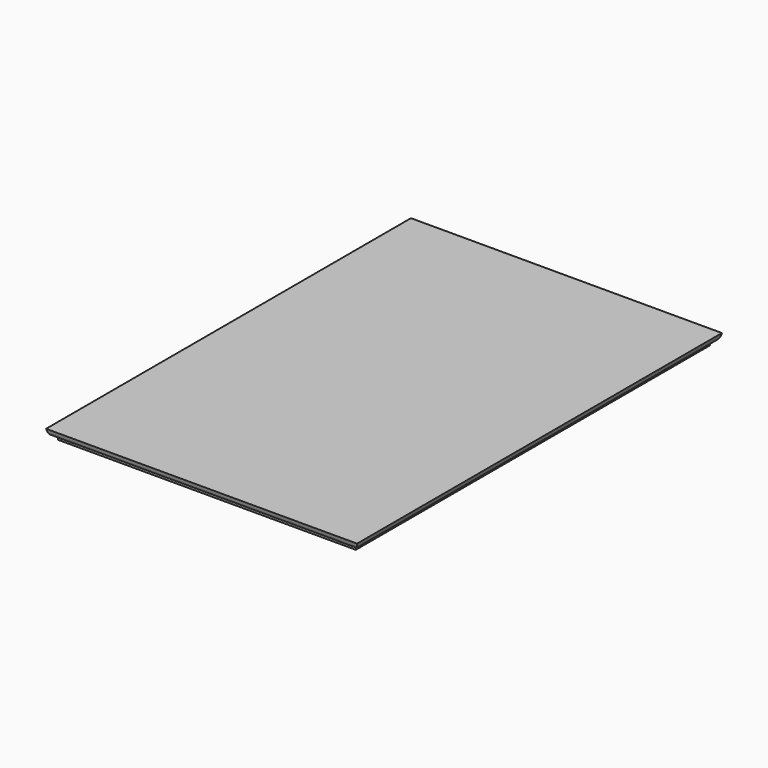
from build123d import *

# Parameters (mm, degrees)
F0_W     = 1524
F0_H     = 2235.2
F1_DEPTH = 50.8
F2_W     = 76.2
F2_H     = 50.8
F3_DEPTH = 12.7
F6_DEPTH = 1524.001
F7_DEPTH = 2235.201


with BuildPart() as f1:
    # F0 (on Top) → F1 (new body)
    with BuildSketch(Plane.XY):
        Rectangle(F0_W, F0_H)
    extrude(amount=F1_DEPTH)

    # F2 (on face) → F3 (cut)
    with BuildSketch(Plane(origin=(0, 0, 0), x_dir=(1, 0, 0), z_dir=(0, 0, -1))):
        with Locations((622.3, 914.4)):
            Rectangle(F2_W, F2_H)
        Polygon((584.2, 939.8), (660.4, 939.8), (660.4, 889), (685.8, 889), (685.8, 990.6), (584.2, 990.6), align=None)
        Polygon((584.2, 889), (584.2, 939.8), (-584.2, 939.8), (-584.2, 889), (-660.4, 889), (-660.4, -889), (-584.2, -889), (-584.2, -939.8), (584.2, -939.8), (584.2, -889), (660.4, -889), (660.4, 889), align=None)
        with Locations((-622.3, 914.4)):
            Rectangle(F2_W, F2_H)
        Polygon((-660.4, 939.8), (-584.2, 939.8), (-584.2, 990.6), (-685.8, 990.6), (-685.8, 889), (-660.4, 889), align=None)
        Polygon((685.8, -889), (660.4, -889), (660.4, -939.8), (584.2, -939.8), (584.2, -990.6), (685.8, -990.6), align=None)
        with Locations((622.3, -914.4)):
            Rectangle(F2_W, F2_H)
        with Locations((-622.3, -914.4)):
            Rectangle(F2_W, F2_H)
        Polygon((-660.4, -939.8), (-660.4, -889), (-685.8, -889), (-685.8, -990.6), (-584.2, -990.6), (-584.2, -939.8), align=None)
    extrude(amount=-F3_DEPTH, mode=Mode.SUBTRACT)

    # F5 (on face) → F6 (cut, through all)
    with BuildSketch(Plane(origin=(-762, 0, 0), x_dir=(0, -1, 0), z_dir=(-1, 0, 0))):
        with BuildLine():
            add(Edge.make_bspline(
                [(-1117.6, 50.8), (-1115.659954, 41.521689), (-1111.224864, 23.411832), (-1093.611323, 16.951729), (-1084.674984, 13.955233)],
                knots=[0, 0, 0, 0, 0.499842, 1, 1, 1, 1], degree=3))
            Line((-1117.6, 50.8), (-1117.6, 0))
            Line((-1117.6, 0), (-1084.674984, 0))
            Line((-1084.674984, 0), (-1084.674984, 13.955233))
        make_face()
        with BuildLine():
            Line((1117.6, 0), (1117.6, 50.8))
            add(Edge.make_bspline(
                [(1117.6, 50.8), (1115.659954, 41.521689), (1111.224864, 23.411832), (1093.611323, 16.951729), (1084.674984, 13.955233)],
                knots=[0, 0, 0, 0, 0.499842, 1, 1, 1, 1], degree=3))
            Line((1084.674984, 13.955233), (1084.674984, 0))
            Line((1084.674984, 0), (1117.6, 0))
        make_face()
    extrude(amount=-F6_DEPTH, mode=Mode.SUBTRACT)

    # F4 (on face) → F7 (cut, through all)
    with BuildSketch(Plane(origin=(0, 1117.6, 0), x_dir=(-1, 0, 0), z_dir=(0, 1, 0))):
        with BuildLine():
            Line((762, 0), (762, 50.8))
            add(Edge.make_bspline(
                [(762, 50.8), (760.054897, 41.497504), (756.173582, 22.935024), (738.306542, 16.943923), (729.393482, 13.955233)],
                knots=[0, 0, 0, 0, 0.501145, 1, 1, 1, 1], degree=3))
            Line((729.393482, 13.955233), (729.393482, 0))
            Line((729.393482, 0), (762, 0))
        make_face()
        with BuildLine():
            add(Edge.make_bspline(
                [(-762, 50.8), (-760.054897, 41.497504), (-756.173582, 22.935024), (-738.306542, 16.943923), (-729.393482, 13.955233)],
                knots=[0, 0, 0, 0, 0.501145, 1, 1, 1, 1], degree=3))
            Line((-762, 50.8), (-762, 0))
            Line((-762, 0), (-729.393482, 0))
            Line((-729.393482, 0), (-729.393482, 13.955233))
        make_face()
    extrude(amount=-F7_DEPTH, mode=Mode.SUBTRACT)


solid = f1.part
